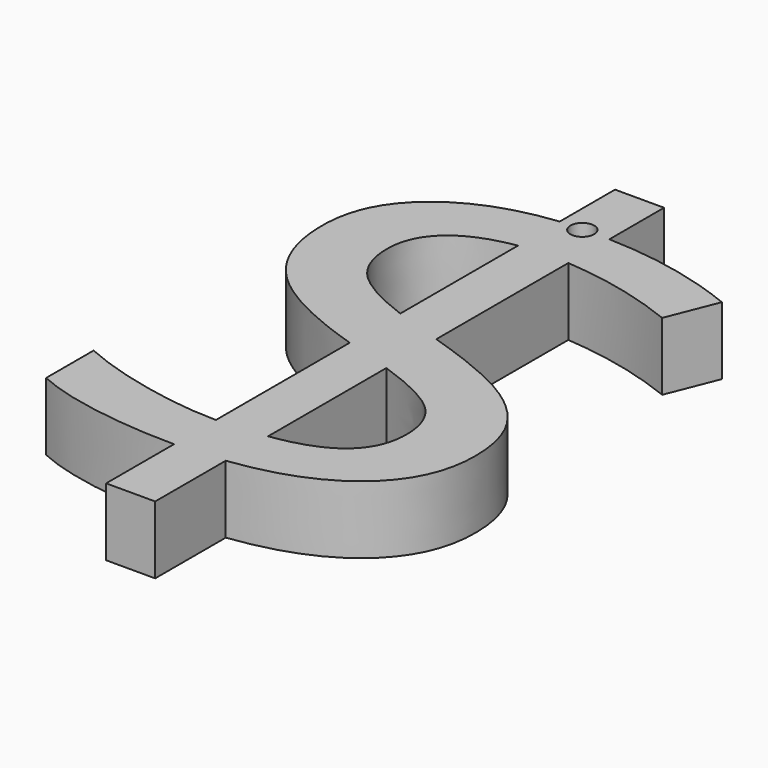
from build123d import *

# Parameters (mm, degrees)
F0_TEXT_SIZE = 58.3989235262
F1_DEPTH     = 5.08
F2_R         = 0.889
F3_DEPTH     = 5.08


# Not quite as in the source:
# - Text() gives the source's letters only with a copy of the font that has no kerning and outlines rounded to 1/6400 em; it was checked with that copy


with BuildPart() as f1:
    # F0 (on Top) → F1 (new body)
    with BuildSketch(Plane.XY):
        with Locations((-33.3330105689, 0)):
            Text('$', F0_TEXT_SIZE, font='Open Sans', text_align=(TextAlign.LEFT, TextAlign.BOTTOM))
    extrude(amount=F1_DEPTH)

    # F2 (on face) → F3 (cut)
    with BuildSketch(Plane.XY.offset(5.08)):
        with Locations((-16.8100813537, 39.1272787626)):
            Circle(F2_R)
    extrude(amount=-F3_DEPTH, mode=Mode.SUBTRACT)


solid = f1.part
